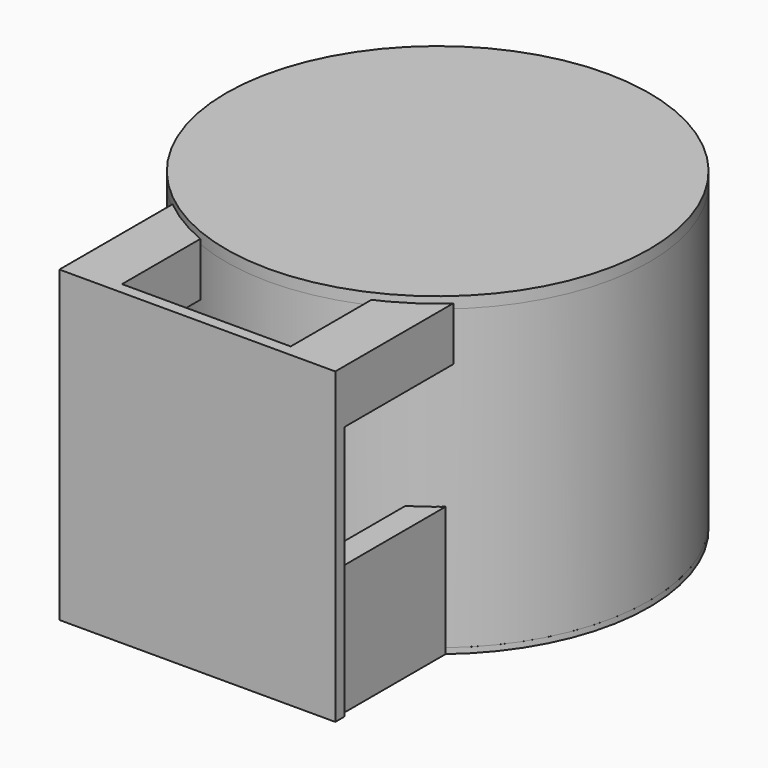
from build123d import *

# Parameters (mm, degrees)
F0_R       = 75
F1_DEPTH   = 105.7
F3_DEPTH   = 148
F4_R       = 2
F5_DEPTH   = 332
F6_W       = 60
F6_H       = 20
F7_DEPTH   = 89
F8_T       = -2.5
F9_R       = 75
F10_DEPTH  = 3
F11_W      = 94.2161493003
F11_H      = 13.6658572592
F12_DEPTH  = 3
F13_R      = 75
F13_R_2    = 2
F14_DEPTH  = 2
F10_FACE_R = 75
F10_FACE_W = 94.2161493003
F10_FACE_H = 13.6658572592
F15_W      = 94.2161493003
F15_H      = 13.6658572592
F16_DEPTH  = 1
F18_DEPTH  = 46
F19_W      = 9
F19_H      = 46
F20_DEPTH  = 4
F21_R      = 5
F22_DEPTH  = 3
F23_W      = 19
F23_H      = 19
F24_DEPTH  = 52.8


with BuildPart() as f1:
    # F0 (on Top) → F1 (new body)
    with BuildSketch(Plane.XY):
        Circle(F0_R)
    extrude(amount=F1_DEPTH)

    # F2 (on face) → F3 (cut)
    with BuildSketch(Plane.XY.offset(105.7)):
        Polygon((49.3204999983, 0), (0, 0), (-48.457699474, 0), (-49.1951782575, -6.9923736234), (48.5333786124, -6.9923736234), align=None)
        Polygon((-48.457699474, 0), (0, 0), (49.3204999983, 0), (50.1076213842, 6.9923736234), (-47.7202206905, 6.9923736234), align=None)
    extrude(amount=-F3_DEPTH, mode=Mode.SUBTRACT)

    # F4 (on face) → F5 (cut)
    with BuildSketch(Plane.XY.offset(105.7)):
        with Locations((-8.4370141849, -49.4647473097)):
            Circle(F4_R)
        with Locations((-64.403899014, 0)):
            Circle(F4_R)
        with Locations((-9.4149308279, 50.376471132)):
            Circle(F4_R)
        with Locations((64.9632513523, 0)):
            Circle(F4_R)
    extrude(amount=-F5_DEPTH, mode=Mode.SUBTRACT)

    # F6 (on face) → F7 (cut)
    with BuildSketch(Plane.XZ.offset(-6.9923736234)):
        with Locations((-11.0256870091, 85)):
            Rectangle(F6_W, F6_H)
    extrude(amount=-F7_DEPTH, mode=Mode.SUBTRACT)

    # F8
    f8_openings = [f1.faces().sort_by_distance(p)[0] for p in [
        (-72.87868, 0, 105.7),
    ]]
    offset(amount=F8_T, openings=f8_openings, kind=Kind.INTERSECTION)


with BuildPart() as f10:
    # F9 (on face) → F10 (new body)
    with BuildSketch(Plane.XY.offset(105.7)):
        Circle(F9_R)
    extrude(amount=F10_DEPTH)

    # F11 (on face) → F12 (cut)
    with BuildSketch(Plane.XY.offset(108.7)):
        with Locations((-2.8760228306, 3.5899474751)):
            Rectangle(F11_W, F11_H)
    extrude(amount=-F12_DEPTH, mode=Mode.SUBTRACT)

    # F10_face (on face) + F15 (on face) → F16 (join)
    with BuildSketch(Plane.XY.offset(108.7)):
        Circle(F10_FACE_R)
        with Locations((-2.8760228306, 3.5899474751)):
            Rectangle(F10_FACE_W, F10_FACE_H, mode=Mode.SUBTRACT)
    with BuildSketch(Plane.XY.offset(108.7)):
        with Locations((-2.8760228306, 3.5899474751)):
            Rectangle(F15_W, F15_H)
    extrude(amount=F16_DEPTH)


with BuildPart() as f14:
    # F13 (on face) → F14 (new body)
    with BuildSketch(Plane(origin=(0, 0, 0), x_dir=(1, 0, 0), z_dir=(0, 0, -1))):
        Circle(F13_R)
        with Locations((-9.4149308279, -50.376471132)):
            Circle(F13_R_2, mode=Mode.SUBTRACT)
        with Locations((-64.403899014, 0)):
            Circle(F13_R_2, mode=Mode.SUBTRACT)
        with Locations((-8.4370141849, 49.4647473097)):
            Circle(F13_R_2, mode=Mode.SUBTRACT)
        Polygon((-49.1951782575, 6.9923736234), (48.5333786124, 6.9923736234), (50.1076213842, -6.9923736234), (-47.7202206905, -6.9923736234), align=None, mode=Mode.SUBTRACT)
        with Locations((64.9632513523, 0)):
            Circle(F13_R_2, mode=Mode.SUBTRACT)
    extrude(amount=F14_DEPTH)

    # F17 (on face) → F18 (join)
    with BuildSketch(Plane(origin=(0, 0, -2), x_dir=(1, 0, 0), z_dir=(0, 0, -1))):
        with BuildLine():
            ThreePointArc((-47.7202206905, 57.8600080993), (-43.3374885628, 61.2116172394), (-38.7202206905, 64.2319586318))
            Line((-38.7202206905, 64.2319586318), (-38.7202206905, 103.9923736234))
            Line((-38.7202206905, 103.9923736234), (-47.7202206905, 103.9923736234))
            Line((-47.7202206905, 103.9923736234), (-47.7202206905, 57.8600080993))
        make_face()
        with BuildLine():
            ThreePointArc((39.5333786124, 63.7346999325), (44.1551881064, 60.6244122717), (48.5333786124, 57.1796393873))
            Line((48.5333786124, 57.1796393873), (48.5333786124, 103.9923736234))
            Line((48.5333786124, 103.9923736234), (39.5333786124, 103.9923736234))
            Line((39.5333786124, 103.9923736234), (39.5333786124, 63.7346999325))
        make_face()
    extrude(amount=-F18_DEPTH)

    # F19 (on face) → F20 (join)
    with BuildSketch(Plane.XZ.offset(103.9923736234)):
        Polygon((-38.7202206905, 44), (-38.7202206905, -2), (50.0812157989, -2), (50.0812157989, 107.3839962482), (-47.7202206905, 107.3839962482), (-47.7202206905, 44), align=None)
        with Locations((-43.2202206905, 21)):
            Rectangle(F19_W, F19_H)
    extrude(amount=F20_DEPTH)

    # F23 (on face) → F24 (join)
    with BuildSketch(Plane(origin=(0, -103.9923736234, 0), x_dir=(-1, 0, 0), z_dir=(0, 1, 0))):
        with Locations((38.2202206905, 97.8839962482)):
            Rectangle(F23_W, F23_H)
        with Locations((-40.5812157989, 97.8839962482)):
            Rectangle(F23_W, F23_H)
    extrude(amount=F24_DEPTH)


with BuildPart() as f22:
    # F21 (on face) → F22 (new body)
    with BuildSketch(Plane(origin=(0, 0, -2), x_dir=(1, 0, 0), z_dir=(0, 0, -1))):
        with Locations((-9.4149308279, -50.376471132)):
            Circle(F21_R)
    extrude(amount=F22_DEPTH)


with BuildPart() as f22b:
    # F21 (on face) → F22, piece 2 (new body)
    with BuildSketch(Plane(origin=(0, 0, -2), x_dir=(1, 0, 0), z_dir=(0, 0, -1))):
        with Locations((64.9632513523, 0)):
            Circle(F21_R)
    extrude(amount=F22_DEPTH)


with BuildPart() as f22c:
    # F21 (on face) → F22, piece 3 (new body)
    with BuildSketch(Plane(origin=(0, 0, -2), x_dir=(1, 0, 0), z_dir=(0, 0, -1))):
        with Locations((-64.403899014, 0)):
            Circle(F21_R)
    extrude(amount=F22_DEPTH)


with BuildPart() as f22d:
    # F21 (on face) → F22, piece 4 (new body)
    with BuildSketch(Plane(origin=(0, 0, -2), x_dir=(1, 0, 0), z_dir=(0, 0, -1))):
        with Locations((-8.4370141849, 49.4647473097)):
            Circle(F21_R)
    extrude(amount=F22_DEPTH)


solid = Compound([f1.part, f10.part, f14.part, f22.part, f22b.part, f22c.part, f22d.part])
